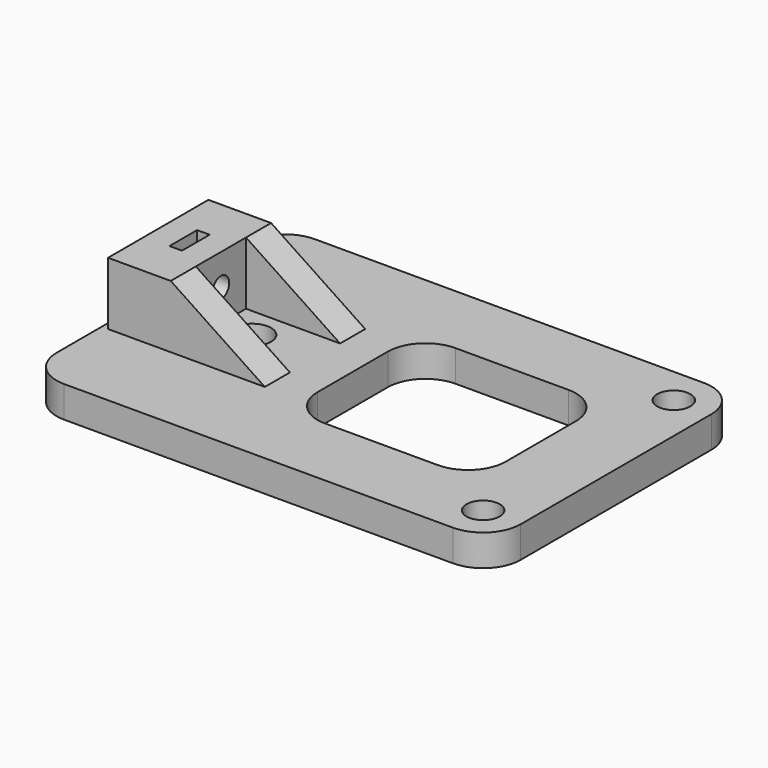
from build123d import *

# Parameters (mm, degrees)
F0_W      = 64
F0_H      = 50
F0_R      = 2.65
F0_R_2    = 3
F1_DEPTH  = 5
F2_W      = 10
F2_H      = 50
F3_DEPTH  = 5
F8_DEPTH  = 10
F10_DEPTH = 35.001
F11_R     = 1.65
F12_DEPTH = 73.001
F15_DEPTH = 1
F16_R     = 6
F17_W     = 30
F17_H     = 26
F18_DEPTH = 5.001
F19_R     = 6


# Not quite as in the source:
# - a feature names something its author has since deleted; it is built from what else it names


with BuildPart() as f1:
    # F0 (on Top) → F1 (new body)
    with BuildSketch(Plane.XY):
        with Locations((32, 25)):
            Rectangle(F0_W, F0_H)
        with Locations((58, 6)):
            Circle(F0_R, mode=Mode.SUBTRACT)
        with Locations((6, 25)):
            Circle(F0_R_2, mode=Mode.SUBTRACT)
        with Locations((58, 44)):
            Circle(F0_R, mode=Mode.SUBTRACT)
    extrude(amount=F1_DEPTH)

    # F2 (on face) → F3 (join, through all)
    with BuildSketch(Plane(origin=(0, 0, 0), x_dir=(1, 0, 0), z_dir=(0, 0, -1))):
        with Locations((-5, -25)):
            Rectangle(F2_W, F2_H)
    extrude(amount=-F3_DEPTH)

    # F16
    f16_edges = [f1.edges().sort_by_distance(p)[0] for p in [
        (64, 50, 2.5),
        (64, 0, 2.5),
        (-10, 0, 2.5),
        (-10, 50, 2.5),
    ]]
    fillet(f16_edges, radius=F16_R)

    # F17 (on face) → F18 (cut, through all)
    with BuildSketch(Plane.XY.offset(5)):
        with Locations((37, 25)):
            Rectangle(F17_W, F17_H)
    extrude(amount=-F18_DEPTH, mode=Mode.SUBTRACT)

    # F19
    f19_edges = [f1.edges().sort_by_distance(p)[0] for p in [
        (22, 38, 2.5),
        (52, 38, 2.5),
        (52, 12, 2.5),
        (22, 12, 2.5),
    ]]
    fillet(f19_edges, radius=F19_R)


with BuildPart() as f8:
    # F7 (on face) → F8 (new body)
    with BuildSketch(Plane.XY.offset(5)):
        Polygon((16, 35), (-9, 35), (-9, 15), (16, 15), (16, 20), (1, 20), (1, 30), (16, 30), align=None)
    extrude(amount=F8_DEPTH)

    # F9 (on face) → F10 (cut, through all)
    with BuildSketch(Plane.XZ.offset(-15)):
        Polygon((16, 15), (1, 15), (16, 5), align=None)
    extrude(amount=-F10_DEPTH, mode=Mode.SUBTRACT)

    # F11 (on face) → F12 (cut, through all)
    with BuildSketch(Plane(origin=(-9, 0, 0), x_dir=(0, -1, 0), z_dir=(-1, 0, 0))):
        with Locations((-25, 10)):
            Circle(F11_R)
    extrude(amount=-F12_DEPTH, mode=Mode.SUBTRACT)

    # F14 (on offset) → F15 (cut, symmetric)
    with BuildSketch(Plane(origin=(-4, 0, 0), x_dir=(0, -1, 0), z_dir=(-1, 0, 0))):
        Polygon((-25, 6.8245735195), (-22.25, 8.4122867597), (-22.25, 15), (-27.75, 15), (-27.75, 8.4122867597), align=None)
    extrude(amount=F15_DEPTH, both=True, mode=Mode.SUBTRACT)


solid = Compound([f1.part, f8.part])
